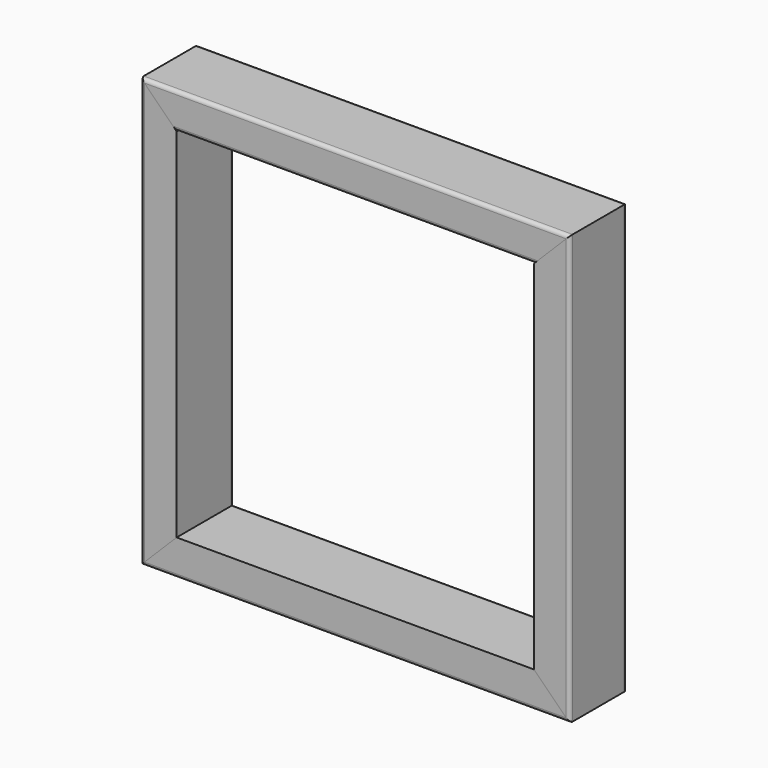
from build123d import *

# Parameters (mm, degrees)
F0_DEPTH = 100
F7_DEPTH = 100
F1_DEPTH = 100
F2_DEPTH = 100
F3_R     = 5
F3_2_R   = 5
F3_3_R   = 5
F4_R     = 5
F8_R     = 5
F5_R     = 5
F5_2_R   = 5
F5_3_R   = 5
F5_4_R   = 5


# Not quite as in the source:
# - a feature names something its author has since deleted; it is built from what else it names


with BuildPart() as f0:
    # F6 (on Front) → F0 (new body)
    with BuildSketch(Plane.XZ):
        Polygon((-635.1203695295, -50), (-585.1203695295, 0), (-1185.1203695295, 0), (-1135.1203695295, -50), align=None)
    extrude(amount=F0_DEPTH)

    # F3
    f3_edges = [f0.edges().sort_by_distance(p)[0] for p in [
        (-885.12037, -100, 0),
        (-885.12037, -100, -50),
    ]]
    fillet(f3_edges, radius=F3_R)

    # F5#2
    f5_2_edges = [f0.edges().sort_by_distance(p)[0] for p in [
        (-885.12037, 0, -50),
        (-885.12037, 0, 0),
    ]]
    fillet(f5_2_edges, radius=F5_2_R)


with BuildPart() as f7:
    # F6 (on Front) → F7 (new body)
    with BuildSketch(Plane.XZ):
        Polygon((-1185.1203695295, 0), (-1185.1203695295, -599.75), (-1184.8703695295, -599.75), (-1135.1203695295, -550), (-1135.1203695295, -50), align=None)
    extrude(amount=F7_DEPTH)

    # F3#2
    f3_2_edges = [f7.edges().sort_by_distance(p)[0] for p in [
        (-1185.12037, -100, -299.875),
    ]]
    fillet(f3_2_edges, radius=F3_2_R)

    # F5#3
    f5_3_edges = [f7.edges().sort_by_distance(p)[0] for p in [
        (-1185.12037, 0, -299.875),
        (-1135.12037, 0, -300),
    ]]
    fillet(f5_3_edges, radius=F5_3_R)


with BuildPart() as f1:
    # F6 (on Front) → F1 (new body)
    with BuildSketch(Plane.XZ):
        Polygon((-1135.1203695295, -600), (-585.1203695295, -600), (-585.1203695295, -599.75), (-635.1203695295, -550), (-1135.1203695295, -550), (-1184.8703695295, -599.75), (-1185.1203695295, -600), align=None)
    extrude(amount=F1_DEPTH)

    # F4
    f4_edges = [f1.edges().sort_by_distance(p)[0] for p in [
        (-885.12037, -100, -600),
    ]]
    fillet(f4_edges, radius=F4_R)

    # F8
    f8_edges = [f1.edges().sort_by_distance(p)[0] for p in [
        (-885.12037, 0, -600),
    ]]
    fillet(f8_edges, radius=F8_R)

    # F5#4
    f5_4_edges = [f1.edges().sort_by_distance(p)[0] for p in [
        (-885.12037, 0, -550),
    ]]
    fillet(f5_4_edges, radius=F5_4_R)


with BuildPart() as f2:
    # F6 (on Front) → F2 (new body)
    with BuildSketch(Plane.XZ):
        Polygon((-635.1203695295, -550), (-585.1203695295, -599.75), (-585.1203695295, 0), (-635.1203695295, -50), align=None)
    extrude(amount=F2_DEPTH)

    # F3#3
    f3_3_edges = [f2.edges().sort_by_distance(p)[0] for p in [
        (-585.12037, -100, -299.875),
    ]]
    fillet(f3_3_edges, radius=F3_3_R)

    # F5
    f5_edges = [f2.edges().sort_by_distance(p)[0] for p in [
        (-585.12037, 0, -299.875),
    ]]
    fillet(f5_edges, radius=F5_R)


solid = Compound([f0.part, f7.part, f1.part, f2.part])
